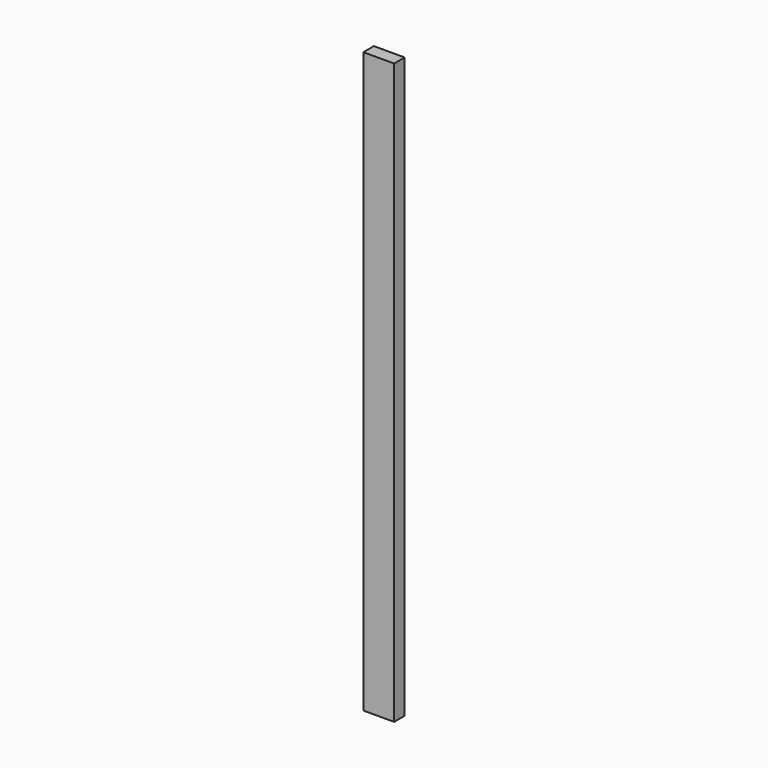
from build123d import *

# Parameters (mm, degrees)
F1_W     = 88.9
F1_H     = 1676.4
F2_DEPTH = 38.1


# Not quite as in the source:
# - a variable given as a bare number and used for a length is read in inches; the dataset says mm whatever the document's units were


with BuildPart() as f2:
    # F1 (on Front) → F2 (new body)
    with BuildSketch(Plane.XZ):
        with Locations((-128.9482451975, 611.4783063787)):
            Rectangle(F1_W, F1_H)
    extrude(amount=F2_DEPTH)


solid = f2.part
